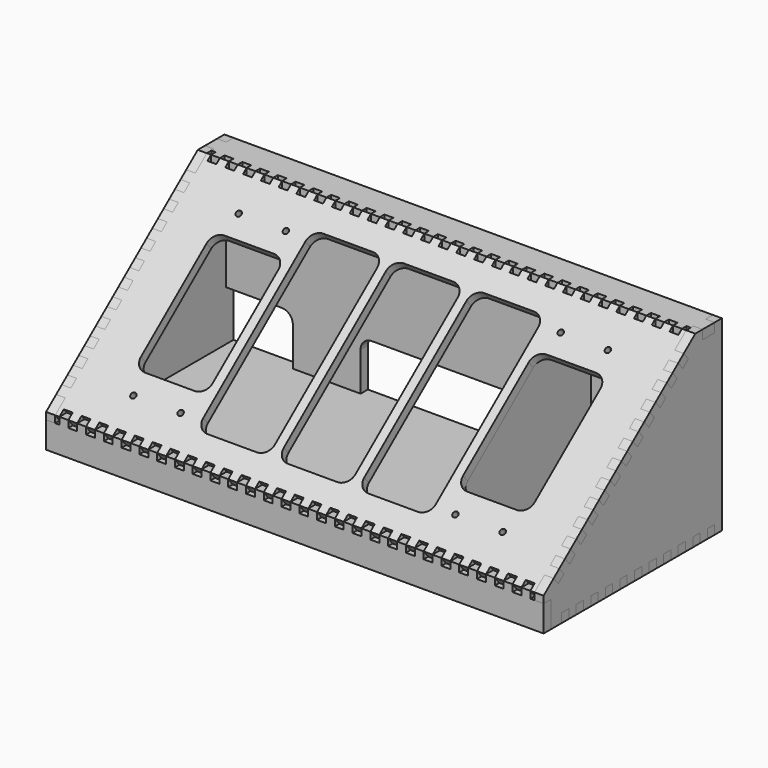
from build123d import *

# Parameters (mm, degrees)
F2_DEPTH       = 142.24
F2_DEPTH_BACK  = 142.24
F3_W           = 5.08
F3_H           = 4.0386
F3_H_2         = 3.2766
F4_DEPTH       = 73.444748786
F5_W           = 5.2
F5_H           = 19.05
F6_DEPTH       = 142.24
F6_DEPTH_BACK  = 142.24
F7_W           = 5.08
F7_H           = 3.9878
F8_DEPTH       = 5.2
F9_W           = 19.05
F9_H           = 5.2
F10_DEPTH      = 142.24
F10_DEPTH_BACK = 142.24
F11_W          = 5.08
F11_H          = 3.2766
F12_DEPTH      = 5.2
F14_DEPTH      = 142.24
F14_DEPTH_BACK = 142.24
F16_DEPTH      = 5.207
F17_W          = 5.207
F17_H          = 5.207
F18_DEPTH      = 5.2
F19_W          = 5.207
F19_H          = 10.5811878652
F19_H_2        = 5.207
F19_H_3        = 9.2456
F20_DEPTH      = 5.2
F21_W          = 5.207
F21_H          = 7.6759982947
F21_H_2        = 5.207
F22_DEPTH      = 5.2
F24_R          = 1.5875
F25_DEPTH      = 5.2
F27_DEPTH      = 5.207
F29_DEPTH      = 5.207


with BuildPart() as f2:
    # F1 (on Right) → F2 (new body, two sides)
    with BuildSketch(Plane.YZ) as f2_sk:
        Polygon((-66.3149991474, 16.45), (-63.0407096173, 12.4103183203), (45.3392886774, 100.2557283862), (42.0649991474, 104.2954100659), align=None)
    extrude(amount=F2_DEPTH)
    extrude(f2_sk.sketch, amount=-F2_DEPTH_BACK)

    # F3 (on face) → F4 (cut, through all)
    with BuildSketch(Plane(origin=(0, -34.3397497185, 42.3669490887), x_dir=(1, 0, 0), z_dir=(0, -0.6296710635, 0.7768618615))):
        with Locations((0, -39.1402046873)):
            Rectangle(F3_W, F3_H)
        with Locations((10.16, -39.1402046873)):
            Rectangle(F3_W, F3_H)
        with Locations((20.32, -39.1402046873)):
            Rectangle(F3_W, F3_H)
        with Locations((30.48, -39.1402046873)):
            Rectangle(F3_W, F3_H)
        with Locations((40.64, -39.1402046873)):
            Rectangle(F3_W, F3_H)
        with Locations((50.8, -39.1402046873)):
            Rectangle(F3_W, F3_H)
        with Locations((60.96, -39.1402046873)):
            Rectangle(F3_W, F3_H)
        with Locations((71.12, -39.1402046873)):
            Rectangle(F3_W, F3_H)
        with Locations((81.28, -39.1402046873)):
            Rectangle(F3_W, F3_H)
        with Locations((91.44, -39.1402046873)):
            Rectangle(F3_W, F3_H)
        with Locations((101.6, -39.1402046873)):
            Rectangle(F3_W, F3_H)
        with Locations((111.76, -39.1402046873)):
            Rectangle(F3_W, F3_H)
        with Locations((121.92, -39.1402046873)):
            Rectangle(F3_W, F3_H)
        with Locations((132.08, -39.1402046873)):
            Rectangle(F3_W, F3_H)
        with Locations((-111.76, -39.1402046873)):
            Rectangle(F3_W, F3_H)
        with Locations((-71.12, -39.1402046873)):
            Rectangle(F3_W, F3_H)
        with Locations((-121.92, -39.1402046873)):
            Rectangle(F3_W, F3_H)
        with Locations((-81.28, -39.1402046873)):
            Rectangle(F3_W, F3_H)
        with Locations((-40.64, -39.1402046873)):
            Rectangle(F3_W, F3_H)
        with Locations((-142.24, -39.1402046873)):
            Rectangle(F3_W, F3_H)
        with Locations((-60.96, -39.1402046873)):
            Rectangle(F3_W, F3_H)
        with Locations((-30.48, -39.1402046873)):
            Rectangle(F3_W, F3_H)
        with Locations((-101.6, -39.1402046873)):
            Rectangle(F3_W, F3_H)
        with Locations((-20.32, -39.1402046873)):
            Rectangle(F3_W, F3_H)
        with Locations((-132.08, -39.1402046873)):
            Rectangle(F3_W, F3_H)
        with Locations((-91.44, -39.1402046873)):
            Rectangle(F3_W, F3_H)
        with Locations((-10.16, -39.1402046873)):
            Rectangle(F3_W, F3_H)
        with Locations((-50.8, -39.1402046873)):
            Rectangle(F3_W, F3_H)
        with Locations((0, 96.7121953127)):
            Rectangle(F3_W, F3_H_2)
        with Locations((142.24, -39.1402046873)):
            Rectangle(F3_W, F3_H)
        with Locations((10.16, 96.7121953127)):
            Rectangle(F3_W, F3_H_2)
        with Locations((20.32, 96.7121953127)):
            Rectangle(F3_W, F3_H_2)
        with Locations((30.48, 96.7121953127)):
            Rectangle(F3_W, F3_H_2)
        with Locations((40.64, 96.7121953127)):
            Rectangle(F3_W, F3_H_2)
        with Locations((50.8, 96.7121953127)):
            Rectangle(F3_W, F3_H_2)
        with Locations((60.96, 96.7121953127)):
            Rectangle(F3_W, F3_H_2)
        with Locations((71.12, 96.7121953127)):
            Rectangle(F3_W, F3_H_2)
        with Locations((81.28, 96.7121953127)):
            Rectangle(F3_W, F3_H_2)
        with Locations((91.44, 96.7121953127)):
            Rectangle(F3_W, F3_H_2)
        with Locations((101.6, 96.7121953127)):
            Rectangle(F3_W, F3_H_2)
        with Locations((111.76, 96.7121953127)):
            Rectangle(F3_W, F3_H_2)
        with Locations((121.92, 96.7121953127)):
            Rectangle(F3_W, F3_H_2)
        with Locations((132.08, 96.7121953127)):
            Rectangle(F3_W, F3_H_2)
        with Locations((142.24, 96.7121953127)):
            Rectangle(F3_W, F3_H_2)
        with Locations((-121.92, 96.7121953127)):
            Rectangle(F3_W, F3_H_2)
        with Locations((-71.12, 96.7121953127)):
            Rectangle(F3_W, F3_H_2)
        with Locations((-81.28, 96.7121953127)):
            Rectangle(F3_W, F3_H_2)
        with Locations((-30.48, 96.7121953127)):
            Rectangle(F3_W, F3_H_2)
        with Locations((-40.64, 96.7121953127)):
            Rectangle(F3_W, F3_H_2)
        with Locations((-91.44, 96.7121953127)):
            Rectangle(F3_W, F3_H_2)
        with Locations((-132.08, 96.7121953127)):
            Rectangle(F3_W, F3_H_2)
        with Locations((-111.76, 96.7121953127)):
            Rectangle(F3_W, F3_H_2)
        with Locations((-20.32, 96.7121953127)):
            Rectangle(F3_W, F3_H_2)
        with Locations((-50.8, 96.7121953127)):
            Rectangle(F3_W, F3_H_2)
        with Locations((-101.6, 96.7121953127)):
            Rectangle(F3_W, F3_H_2)
        with Locations((-10.16, 96.7121953127)):
            Rectangle(F3_W, F3_H_2)
        with Locations((-60.96, 96.7121953127)):
            Rectangle(F3_W, F3_H_2)
        with Locations((-142.24, 96.7121953127)):
            Rectangle(F3_W, F3_H_2)
    extrude(amount=-F4_DEPTH, mode=Mode.SUBTRACT)


with BuildPart() as f6:
    # F5 (on Right) → F6 (new body, two sides)
    with BuildSketch(Plane.YZ) as f6_sk:
        with Locations((-63.7149991474, 6.925)):
            Rectangle(F5_W, F5_H)
    extrude(amount=F6_DEPTH)
    extrude(f6_sk.sketch, amount=-F6_DEPTH_BACK)

    # F7 (on face) → F8 (cut, through all)
    with BuildSketch(Plane.XZ.offset(66.3149991474)):
        with Locations((5.08, 14.4561)):
            Rectangle(F7_W, F7_H)
        with Locations((15.24, 14.4561)):
            Rectangle(F7_W, F7_H)
        with Locations((25.4, 14.4561)):
            Rectangle(F7_W, F7_H)
        with Locations((35.56, 14.4561)):
            Rectangle(F7_W, F7_H)
        with Locations((45.72, 14.4561)):
            Rectangle(F7_W, F7_H)
        with Locations((55.88, 14.4561)):
            Rectangle(F7_W, F7_H)
        with Locations((66.04, 14.4561)):
            Rectangle(F7_W, F7_H)
        with Locations((76.2, 14.4561)):
            Rectangle(F7_W, F7_H)
        with Locations((86.36, 14.4561)):
            Rectangle(F7_W, F7_H)
        with Locations((96.52, 14.4561)):
            Rectangle(F7_W, F7_H)
        with Locations((106.68, 14.4561)):
            Rectangle(F7_W, F7_H)
        with Locations((116.84, 14.4561)):
            Rectangle(F7_W, F7_H)
        with Locations((127, 14.4561)):
            Rectangle(F7_W, F7_H)
        Polygon((139.7, 16.45), (134.62, 16.45), (134.62, 12.4622), (139.7, 12.4622), (142.24, 12.4622), (142.24, 16.45), align=None)
        with Locations((-5.08, 14.4561)):
            Rectangle(F7_W, F7_H)
        Polygon((-139.7, 12.4622), (-134.62, 12.4622), (-134.62, 16.45), (-139.7, 16.45), (-142.24, 16.45), (-142.24, 12.4622), align=None)
        with Locations((-55.88, 14.4561)):
            Rectangle(F7_W, F7_H)
        with Locations((-96.52, 14.4561)):
            Rectangle(F7_W, F7_H)
        with Locations((-35.56, 14.4561)):
            Rectangle(F7_W, F7_H)
        with Locations((-76.2, 14.4561)):
            Rectangle(F7_W, F7_H)
        with Locations((-116.84, 14.4561)):
            Rectangle(F7_W, F7_H)
        with Locations((-66.04, 14.4561)):
            Rectangle(F7_W, F7_H)
        with Locations((-106.68, 14.4561)):
            Rectangle(F7_W, F7_H)
        with Locations((-45.72, 14.4561)):
            Rectangle(F7_W, F7_H)
        with Locations((-86.36, 14.4561)):
            Rectangle(F7_W, F7_H)
        with Locations((-127, 14.4561)):
            Rectangle(F7_W, F7_H)
        with Locations((-25.4, 14.4561)):
            Rectangle(F7_W, F7_H)
        with Locations((-15.24, 14.4561)):
            Rectangle(F7_W, F7_H)
    extrude(amount=-F8_DEPTH, mode=Mode.SUBTRACT)


with BuildPart() as f10:
    # F9 (on Right) → F10 (new body, two sides)
    with BuildSketch(Plane.YZ) as f10_sk:
        with Locations((51.5899991474, 101.6954100659)):
            Rectangle(F9_W, F9_H)
    extrude(amount=F10_DEPTH)
    extrude(f10_sk.sketch, amount=-F10_DEPTH_BACK)

    # F11 (on face) → F12 (cut, through all)
    with BuildSketch(Plane.XY.offset(104.2954100659)):
        with Locations((5.08, 43.7032991474)):
            Rectangle(F11_W, F11_H)
        with Locations((-5.08, 43.7032991474)):
            Rectangle(F11_W, F11_H)
        with Locations((15.24, 43.7032991474)):
            Rectangle(F11_W, F11_H)
        with Locations((25.4, 43.7032991474)):
            Rectangle(F11_W, F11_H)
        with Locations((35.56, 43.7032991474)):
            Rectangle(F11_W, F11_H)
        with Locations((45.72, 43.7032991474)):
            Rectangle(F11_W, F11_H)
        with Locations((55.88, 43.7032991474)):
            Rectangle(F11_W, F11_H)
        with Locations((66.04, 43.7032991474)):
            Rectangle(F11_W, F11_H)
        with Locations((76.2, 43.7032991474)):
            Rectangle(F11_W, F11_H)
        with Locations((86.36, 43.7032991474)):
            Rectangle(F11_W, F11_H)
        with Locations((96.52, 43.7032991474)):
            Rectangle(F11_W, F11_H)
        with Locations((106.68, 43.7032991474)):
            Rectangle(F11_W, F11_H)
        with Locations((116.84, 43.7032991474)):
            Rectangle(F11_W, F11_H)
        with Locations((127, 43.7032991474)):
            Rectangle(F11_W, F11_H)
        with Locations((137.16, 43.7032991474)):
            Rectangle(F11_W, F11_H)
        with Locations((-86.36, 43.7032991474)):
            Rectangle(F11_W, F11_H)
        with Locations((-106.68, 43.7032991474)):
            Rectangle(F11_W, F11_H)
        with Locations((-35.56, 43.7032991474)):
            Rectangle(F11_W, F11_H)
        with Locations((-96.52, 43.7032991474)):
            Rectangle(F11_W, F11_H)
        with Locations((-55.88, 43.7032991474)):
            Rectangle(F11_W, F11_H)
        with Locations((-137.16, 43.7032991474)):
            Rectangle(F11_W, F11_H)
        with Locations((-116.84, 43.7032991474)):
            Rectangle(F11_W, F11_H)
        with Locations((-66.04, 43.7032991474)):
            Rectangle(F11_W, F11_H)
        with Locations((-76.2, 43.7032991474)):
            Rectangle(F11_W, F11_H)
        with Locations((-127, 43.7032991474)):
            Rectangle(F11_W, F11_H)
        with Locations((-15.24, 43.7032991474)):
            Rectangle(F11_W, F11_H)
        with Locations((-45.72, 43.7032991474)):
            Rectangle(F11_W, F11_H)
        with Locations((-25.4, 43.7032991474)):
            Rectangle(F11_W, F11_H)
    extrude(amount=-F12_DEPTH, mode=Mode.SUBTRACT)


with BuildPart() as f14:
    # F13 (on Right) → F14 (new body, two sides)
    with BuildSketch(Plane.YZ) as f14_sk:
        Polygon((-61.1149991474, 2.6), (-61.1149991474, -2.6), (61.1149991474, -2.6), (61.1149991474, 2.6), (55.9149991474, 2.6), align=None)
    extrude(amount=F14_DEPTH)
    extrude(f14_sk.sketch, amount=-F14_DEPTH_BACK)

    # F21 (on face) → F22 (cut, through all)
    with BuildSketch(Plane(origin=(0, 0, -2.6), x_dir=(1, 0, 0), z_dir=(0, 0, -1))):
        with Locations((139.6365, 57.277)):
            Rectangle(F21_W, F21_H)
        with Locations((139.6365, 45.6285008526)):
            Rectangle(F21_W, F21_H_2)
        with Locations((139.6365, 35.2145008526)):
            Rectangle(F21_W, F21_H_2)
        with Locations((139.6365, 24.8005008526)):
            Rectangle(F21_W, F21_H_2)
        with Locations((139.6365, 14.3865008526)):
            Rectangle(F21_W, F21_H_2)
        with Locations((139.6365, 3.9725008526)):
            Rectangle(F21_W, F21_H_2)
        with Locations((139.6365, -6.4414991474)):
            Rectangle(F21_W, F21_H_2)
        with Locations((139.6365, -16.8554991474)):
            Rectangle(F21_W, F21_H_2)
        with Locations((139.6365, -27.2694991474)):
            Rectangle(F21_W, F21_H_2)
        with Locations((139.6365, -37.6834991474)):
            Rectangle(F21_W, F21_H_2)
        with Locations((139.6365, -48.0974991474)):
            Rectangle(F21_W, F21_H_2)
        with Locations((139.6365, -58.5114991474)):
            Rectangle(F21_W, F21_H_2)
        with Locations((-139.6365, -6.4414991474)):
            Rectangle(F21_W, F21_H_2)
        with Locations((-139.6365, 45.6285008526)):
            Rectangle(F21_W, F21_H_2)
        with Locations((-139.6365, 14.3865008526)):
            Rectangle(F21_W, F21_H_2)
        with Locations((-139.6365, -16.8554991474)):
            Rectangle(F21_W, F21_H_2)
        with Locations((-139.6365, -27.2694991474)):
            Rectangle(F21_W, F21_H_2)
        with Locations((-139.6365, -58.5114991474)):
            Rectangle(F21_W, F21_H_2)
        with Locations((-139.6365, -37.6834991474)):
            Rectangle(F21_W, F21_H_2)
        with Locations((-139.6365, 3.9725008526)):
            Rectangle(F21_W, F21_H_2)
        with Locations((-139.6365, 24.8005008526)):
            Rectangle(F21_W, F21_H_2)
        with Locations((-139.6365, 35.2145008526)):
            Rectangle(F21_W, F21_H_2)
        with Locations((-139.6365, -48.0974991474)):
            Rectangle(F21_W, F21_H_2)
        with Locations((-139.6365, 57.277)):
            Rectangle(F21_W, F21_H)
    extrude(amount=-F22_DEPTH, mode=Mode.SUBTRACT)


with BuildPart() as f16:
    # F15 (on face) → F16 (new body)
    with BuildSketch(Plane.YZ.offset(142.24)):
        Polygon((-59.1324451209, 22.2716867845), (-66.3149991474, 16.45), (-66.3149991474, 12.4622), (-61.1149991474, 12.4622), (-61.1149991474, -2.6), (-53.4390008526, -2.6), (-53.4390008526, 2.6), (-48.2320008526, 2.6), (-48.2320008526, -2.6), (-43.0250008526, -2.6), (-43.0250008526, 2.6), (-37.8180008526, 2.6), (-37.8180008526, -2.6), (-32.6110008526, -2.6), (-32.6110008526, 2.6), (-27.4040008526, 2.6), (-27.4040008526, -2.6), (-22.1970008526, -2.6), (-22.1970008526, 2.6), (-16.9900008526, 2.6), (-16.9900008526, -2.6), (-11.7830008526, -2.6), (-11.7830008526, 2.6), (-6.5760008526, 2.6), (-6.5760008526, -2.6), (-1.3690008526, -2.6), (-1.3690008526, 2.6), (3.8379991474, 2.6), (3.8379991474, -2.6), (9.0449991474, -2.6), (9.0449991474, 2.6), (14.2519991474, 2.6), (14.2519991474, -2.6), (19.4589991474, -2.6), (19.4589991474, 2.6), (24.6659991474, 2.6), (24.6659991474, -2.6), (29.8729991474, -2.6), (29.8729991474, 2.6), (35.0799991474, 2.6), (35.0799991474, -2.6), (40.2869991474, -2.6), (40.2869991474, 2.6), (45.4939991474, 2.6), (45.4939991474, -2.6), (50.7009991474, -2.6), (50.7009991474, 2.6), (55.9079991474, 2.6), (55.9079991474, -2.6), (61.1149991474, -2.6), (61.1149991474, 104.2954100659), (55.9079991474, 104.2954100659), (55.9079991474, 99.0954100659), (47.2719991474, 99.0954100659), (47.2719991474, 104.2954100659), (42.0649991474, 104.2954100659), (33.8448778457, 97.6327422499), (37.1191673758, 93.5930605702), (33.0795413382, 90.3188161398), (29.8052518081, 94.3584978194), (25.7601320954, 91.0798005919), (29.0344216255, 87.0401189122), (24.9947955878, 83.7658744818), (21.7205060577, 87.8055561614), (17.675386345, 84.5268589339), (20.9496758751, 80.4871772542), (16.9100498375, 77.2129328238), (13.6357603074, 81.2526145035), (9.5906405947, 77.9739172759), (12.8649301248, 73.9342355962), (8.8253040871, 70.6599911658), (5.551014557, 74.6996728455), (1.5058948443, 71.4209756179), (4.7801843744, 67.3812939383), (0.7405583368, 64.1070495078), (-2.5337311933, 68.1467311875), (-6.578850906, 64.86803396), (-3.304561376, 60.8283522803), (-7.3441874136, 57.5541078498), (-10.6184769437, 61.5937895295), (-14.6635966564, 58.315092302), (-11.3893071263, 54.2754106223), (-15.428933164, 51.0011661918), (-18.703222694, 55.0408478715), (-22.7483424068, 51.762150644), (-19.4740528767, 47.7224689643), (-23.5136789143, 44.4482245338), (-26.7879684444, 48.4879062135), (-30.8330881571, 45.209208986), (-27.558798627, 41.1695273063), (-31.5984246647, 37.8952828759), (-34.8727141947, 41.9349645555), (-38.9178339075, 38.656267328), (-35.6435443774, 34.6165856483), (-39.683170415, 31.3423412179), (-42.9574599451, 35.3820228975), (-47.0025796578, 32.10332567), (-43.7282901277, 28.0636439903), (-47.7679161654, 24.7893995599), (-51.0422056955, 28.8290812396), (-55.0873254082, 25.550384012), (-51.8130358781, 21.5107023323), (-55.8581555908, 18.2320051048), align=None)
    extrude(amount=-F16_DEPTH)


with BuildPart() as f18_tool:
    # F17 (on face) → F18 (new body, through all)
    with BuildSketch(Plane.XY.offset(104.2954100659)):
        with Locations((139.6365, 58.5114991474)):
            Rectangle(F17_W, F17_H)
        with Locations((139.6365, 44.6684991474)):
            Rectangle(F17_W, F17_H)
        with Locations((-139.6365, 58.5114991474)):
            Rectangle(F17_W, F17_H)
        with Locations((-139.6365, 44.6684991474)):
            Rectangle(F17_W, F17_H)
    extrude(amount=-F18_DEPTH)


with BuildPart() as f2_1:
    add(f2.part)

    # F18: cut by f18_tool
    add(f18_tool.part, mode=Mode.SUBTRACT)

    # F19 (on face) → F20 (cut, through all)
    with BuildSketch(Plane(origin=(0, -34.3397497185, 42.3669490887), x_dir=(1, 0, 0), z_dir=(0, -0.6296710635, 0.7768618615))):
        with Locations((139.6365, 93.0599013801)):
            Rectangle(F19_W, F19_H)
        with Locations((139.6365, 79.9658790716)):
            Rectangle(F19_W, F19_H_2)
        with Locations((139.6365, 69.5589506957)):
            Rectangle(F19_W, F19_H_2)
        with Locations((139.6365, 59.1520223198)):
            Rectangle(F19_W, F19_H_2)
        with Locations((139.6365, 48.7450939439)):
            Rectangle(F19_W, F19_H_2)
        with Locations((139.6365, 38.3381655681)):
            Rectangle(F19_W, F19_H_2)
        with Locations((139.6365, 27.9312371922)):
            Rectangle(F19_W, F19_H_2)
        with Locations((139.6365, 17.5243088163)):
            Rectangle(F19_W, F19_H_2)
        with Locations((139.6365, 7.1173804404)):
            Rectangle(F19_W, F19_H_2)
        with Locations((139.6365, -3.2895479355)):
            Rectangle(F19_W, F19_H_2)
        with Locations((139.6365, -13.6964763114)):
            Rectangle(F19_W, F19_H_2)
        with Locations((139.6365, -24.1034046873)):
            Rectangle(F19_W, F19_H_2)
        with Locations((139.6365, -36.5367046873)):
            Rectangle(F19_W, F19_H_3)
        with Locations((-139.6365, 17.5243088163)):
            Rectangle(F19_W, F19_H_2)
        with Locations((-139.6365, 79.9658790716)):
            Rectangle(F19_W, F19_H_2)
        with Locations((-139.6365, 7.1173804404)):
            Rectangle(F19_W, F19_H_2)
        with Locations((-139.6365, 48.7450939439)):
            Rectangle(F19_W, F19_H_2)
        with Locations((-139.6365, -3.2895479355)):
            Rectangle(F19_W, F19_H_2)
        with Locations((-139.6365, -24.1034046873)):
            Rectangle(F19_W, F19_H_2)
        with Locations((-139.6365, 27.9312371922)):
            Rectangle(F19_W, F19_H_2)
        with Locations((-139.6365, 69.5589506957)):
            Rectangle(F19_W, F19_H_2)
        with Locations((-139.6365, 38.3381655681)):
            Rectangle(F19_W, F19_H_2)
        with Locations((-139.6365, 59.1520223198)):
            Rectangle(F19_W, F19_H_2)
        with Locations((-139.6365, -13.6964763114)):
            Rectangle(F19_W, F19_H_2)
        with Locations((-139.6365, 93.0599013801)):
            Rectangle(F19_W, F19_H)
        with Locations((-139.6365, -36.5367046873)):
            Rectangle(F19_W, F19_H_3)
    extrude(amount=-F20_DEPTH, mode=Mode.SUBTRACT)

    # F24 (on face) → F25 (cut, through all)
    with BuildSketch(Plane(origin=(0, -34.3397497185, 42.3669490887), x_dir=(1, 0, 0), z_dir=(0, -0.6296710635, 0.7768618615))):
        with BuildLine():
            Line((-14.15, -24.7445046873), (14.15, -24.7445046873))
            ThreePointArc((14.15, -24.7445046873), (18.6401280605, -22.8846327478), (20.5, -18.3945046873))
            Line((20.5, -18.3945046873), (20.5, 75.5854953127))
            ThreePointArc((20.5, 75.5854953127), (18.6401280605, 80.0756233733), (14.15, 81.9354953127))
            Line((14.15, 81.9354953127), (-14.15, 81.9354953127))
            ThreePointArc((-14.15, 81.9354953127), (-18.6401280605, 80.0756233733), (-20.5, 75.5854953127))
            Line((-20.5, 75.5854953127), (-20.5, -18.3945046873))
            ThreePointArc((-20.5, -18.3945046873), (-18.6401280605, -22.8846327478), (-14.15, -24.7445046873))
        make_face()
        with BuildLine():
            ThreePointArc((66.5375, 75.5854953127), (64.6776280605, 80.0756233733), (60.1875, 81.9354953127))
            Line((60.1875, 81.9354953127), (31.8875, 81.9354953127))
            ThreePointArc((31.8875, 81.9354953127), (27.3973719395, 80.0756233733), (25.5375, 75.5854953127))
            Line((25.5375, 75.5854953127), (25.5375, -18.3945046873))
            ThreePointArc((25.5375, -18.3945046873), (27.3973719395, -22.8846327478), (31.8875, -24.7445046873))
            Line((31.8875, -24.7445046873), (60.1875, -24.7445046873))
            ThreePointArc((60.1875, -24.7445046873), (64.6776280605, -22.8846327478), (66.5375, -18.3945046873))
            Line((66.5375, -18.3945046873), (66.5375, 75.5854953127))
        make_face()
        with BuildLine():
            ThreePointArc((106.225, -7.9170046873), (110.7151280605, -6.0571327478), (112.575, -1.5670046873))
            Line((112.575, -1.5670046873), (112.575, 58.7579953127))
            ThreePointArc((112.575, 58.7579953127), (110.7151280605, 63.2481233733), (106.225, 65.1079953127))
            Line((106.225, 65.1079953127), (77.925, 65.1079953127))
            ThreePointArc((77.925, 65.1079953127), (73.4348719395, 63.2481233733), (71.575, 58.7579953127))
            Line((71.575, 58.7579953127), (71.575, -1.5670046873))
            ThreePointArc((71.575, -1.5670046873), (73.4348719395, -6.0571327478), (77.925, -7.9170046873))
            Line((77.925, -7.9170046873), (106.225, -7.9170046873))
        make_face()
        with Locations((78.58125, 77.0142453127)):
            Circle(F24_R)
        with Locations((105.56875, 77.0142453127)):
            Circle(F24_R)
        with Locations((105.56875, -19.8232546873)):
            Circle(F24_R)
        with Locations((78.58125, -19.8232546873)):
            Circle(F24_R)
        with BuildLine():
            ThreePointArc((-71.575, 58.7579953127), (-73.4348719395, 63.2481233733), (-77.925, 65.1079953127))
            Line((-77.925, 65.1079953127), (-106.225, 65.1079953127))
            ThreePointArc((-106.225, 65.1079953127), (-110.7151280605, 63.2481233733), (-112.575, 58.7579953127))
            Line((-112.575, 58.7579953127), (-112.575, -1.5670046873))
            ThreePointArc((-112.575, -1.5670046873), (-110.7151280605, -6.0571327478), (-106.225, -7.9170046873))
            Line((-106.225, -7.9170046873), (-77.925, -7.9170046873))
            ThreePointArc((-77.925, -7.9170046873), (-73.4348719395, -6.0571327478), (-71.575, -1.5670046873))
            Line((-71.575, -1.5670046873), (-71.575, 58.7579953127))
        make_face()
        with Locations((-78.58125, 77.0142453127)):
            Circle(F24_R)
        with Locations((-78.58125, -19.8232546873)):
            Circle(F24_R)
        with Locations((-105.56875, 77.0142453127)):
            Circle(F24_R)
        with Locations((-105.56875, -19.8232546873)):
            Circle(F24_R)
        with BuildLine():
            Line((-31.8875, 81.9354953127), (-60.1875, 81.9354953127))
            ThreePointArc((-60.1875, 81.9354953127), (-64.6776280605, 80.0756233733), (-66.5375, 75.5854953127))
            Line((-66.5375, 75.5854953127), (-66.5375, -18.3945046873))
            ThreePointArc((-66.5375, -18.3945046873), (-64.6776280605, -22.8846327478), (-60.1875, -24.7445046873))
            Line((-60.1875, -24.7445046873), (-31.8875, -24.7445046873))
            ThreePointArc((-31.8875, -24.7445046873), (-27.3973719395, -22.8846327478), (-25.5375, -18.3945046873))
            Line((-25.5375, -18.3945046873), (-25.5375, 75.5854953127))
            ThreePointArc((-25.5375, 75.5854953127), (-27.3973719395, 80.0756233733), (-31.8875, 81.9354953127))
        make_face()
    extrude(amount=-F25_DEPTH, mode=Mode.SUBTRACT)


with BuildPart() as f10_1:
    add(f10.part)

    # F18: cut by f18_tool
    add(f18_tool.part, mode=Mode.SUBTRACT)


with BuildPart() as f23_1:
    # F23: copy of F16
    add(f16.part.moved(Location((-279.273, 0, 0))))


with BuildPart() as f27:
    # F26 (on face) → F27 (new body)
    with BuildSketch(Plane.YZ.offset(71.575)):
        Polygon((-45.2399991474, 2.6), (55.9149991474, 2.6), (55.9149991474, 99.0954100659), (43.9077363916, 99.0954100659), (-45.2399991474, 26.8383561068), align=None)
    extrude(amount=-F27_DEPTH)


with BuildPart() as f29:
    # F28 (on face) → F29 (new body)
    with BuildSketch(Plane(origin=(0, 61.1149991474, 0), x_dir=(-1, 0, 0), z_dir=(0, 1, 0))):
        with BuildLine():
            Line((137.033, 99.0954100659), (-137.033, 99.0954100659))
            Line((-137.033, 99.0954100659), (-137.033, 31.175))
            Line((-137.033, 31.175), (-105.283, 31.175))
            ThreePointArc((-105.283, 31.175), (-100.7928719395, 29.3151280605), (-98.933, 24.825))
            Line((-98.933, 24.825), (-98.933, 2.6))
            Line((-98.933, 2.6), (-60.1875, 2.6))
            Line((-60.1875, 2.6), (-60.1875, 24.825))
            ThreePointArc((-60.1875, 24.825), (-58.3276280605, 29.3151280605), (-53.8375, 31.175))
            Line((-53.8375, 31.175), (53.8375, 31.175))
            ThreePointArc((53.8375, 31.175), (58.3276280605, 29.3151280605), (60.1875, 24.825))
            Line((60.1875, 24.825), (60.1875, 2.6))
            Line((60.1875, 2.6), (98.933, 2.6))
            Line((98.933, 2.6), (98.933, 24.825))
            ThreePointArc((98.933, 24.825), (100.7928719395, 29.3151280605), (105.283, 31.175))
            Line((105.283, 31.175), (137.033, 31.175))
            Line((137.033, 31.175), (137.033, 99.0954100659))
        make_face()
    extrude(amount=-F29_DEPTH)


solid = Compound([f6.part, f14.part, f16.part, f2_1.part, f10_1.part, f23_1.part, f27.part, f29.part])
